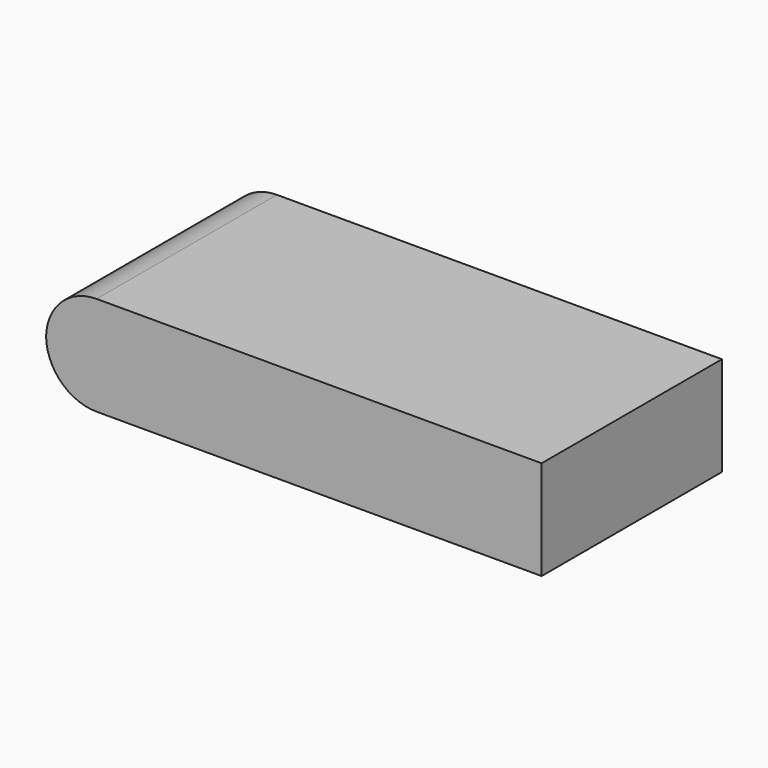
from build123d import *

# Parameters (mm, degrees)
F0_W        = 71.6
F0_H        = 14.35
F1_DEPTH    = 32.56
F2_T1_DEPTH = 69.06


# Not quite as in the source:
# - a fillet or chamfer that OpenCascade refuses, or shapes differently, is made with other operations: its cross-section is extruded or revolved along the edge and cut away or added


with BuildPart() as f1:
    # F0 (on Front) → F1 (new body)
    with BuildSketch(Plane.XZ):
        Rectangle(F0_W, F0_H)
    extrude(amount=F1_DEPTH)

    # F2: fillet of radius 7.3 on 2 edges, made by hand

    # F2_s2 → F2_t1 (cut)
    with BuildSketch(Plane.XZ.offset(-18.25)):
        with BuildLine():
            ThreePointArc((-28.5, 7.175), (-33.6618795027, 5.0368795027), (-35.8, -0.125))
            Line((-35.8, -0.125), (-35.8, 7.175))
            Line((-35.8, 7.175), (-28.5, 7.175))
        make_face()
        with BuildLine():
            ThreePointArc((-35.8, 0.125), (-33.6618795027, -5.0368795027), (-28.5, -7.175))
            Line((-28.5, -7.175), (-35.8, -7.175))
            Line((-35.8, -7.175), (-35.8, 0.125))
        make_face()
    extrude(amount=F2_T1_DEPTH, mode=Mode.SUBTRACT)


solid = f1.part
